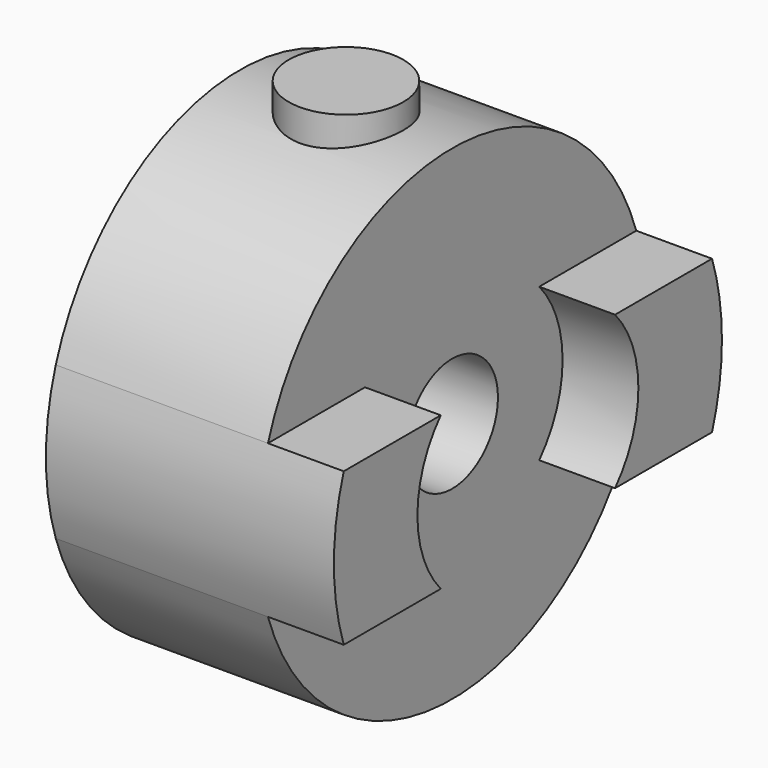
from build123d import *

# Parameters (mm, degrees)
F0_R     = 1.5
F1_DEPTH = 5.55625
F2_DEPTH = 1.984375
F3_R     = 1.5
F4_DEPTH = 7


# Not quite as in the source:
# - a length typed as a fraction of an inch, garbled in the dataset ("3 / 203.2 mm" for 3/8 in), is restored


with BuildPart() as f1:
    # F0 (on Right) → F1 (new body)
    with BuildSketch(Plane.YZ):
        with BuildLine():
            Line((2.851815, 2), (6.026815, 2))
            ThreePointArc((6.026815, 2), (0, 6.35), (-6.026815, 2))
            Line((-6.026815, 2), (-2.851815, 2))
            ThreePointArc((-2.851815, 2), (-3.615747, 0), (-2.851815, -2))
            Line((-2.851815, -2), (-6.026815, -2))
            ThreePointArc((-6.026815, -2), (0, -6.35), (6.026815, -2))
            Line((6.026815, -2), (2.851815, -2))
            ThreePointArc((2.851815, -2), (3.615747, 0), (2.851815, 2))
        make_face()
        Circle(F0_R, mode=Mode.SUBTRACT)
        with BuildLine():
            Line((-2.851815, 2), (-6.026815, 2))
            ThreePointArc((-6.026815, 2), (-6.35, 0), (-6.026815, -2))
            Line((-6.026815, -2), (-2.851815, -2))
            ThreePointArc((-2.851815, -2), (-3.615747, 0), (-2.851815, 2))
        make_face()
        with BuildLine():
            ThreePointArc((6.026815, -2), (6.268683, -1.012972), (6.35, 0))
            ThreePointArc((6.35, 0), (6.268683, 1.012972), (6.026815, 2))
            Line((6.026815, 2), (2.851815, 2))
            ThreePointArc((2.851815, 2), (3.615747, 0), (2.851815, -2))
            Line((2.851815, -2), (6.026815, -2))
        make_face()
    extrude(amount=-F1_DEPTH)

    # F0 (on Right) → F2 (join)
    with BuildSketch(Plane.YZ):
        with BuildLine():
            Line((-2.851815, 2), (-6.026815, 2))
            ThreePointArc((-6.026815, 2), (-6.35, 0), (-6.026815, -2))
            Line((-6.026815, -2), (-2.851815, -2))
            ThreePointArc((-2.851815, -2), (-3.615747, 0), (-2.851815, 2))
        make_face()
        with BuildLine():
            ThreePointArc((6.026815, -2), (6.268683, -1.012972), (6.35, 0))
            ThreePointArc((6.35, 0), (6.268683, 1.012972), (6.026815, 2))
            Line((6.026815, 2), (2.851815, 2))
            ThreePointArc((2.851815, 2), (3.615747, 0), (2.851815, -2))
            Line((2.851815, -2), (6.026815, -2))
        make_face()
    extrude(amount=F2_DEPTH)

    # F3 (on Top) → F4 (join)
    with BuildSketch(Plane.XY):
        with Locations((-2.778125, 0)):
            Circle(F3_R)
    extrude(amount=F4_DEPTH)


solid = f1.part
